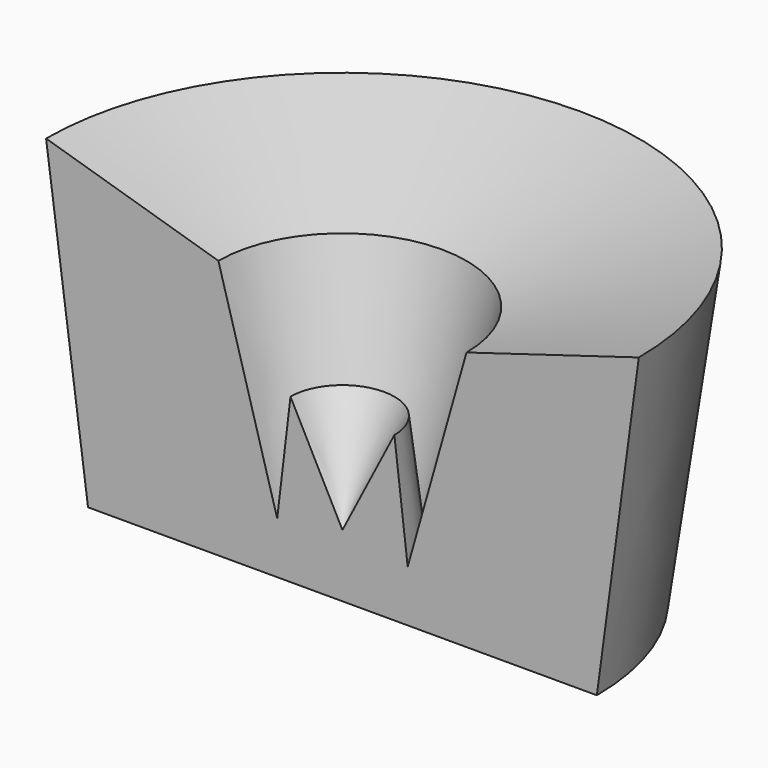
from build123d import *

# Parameters (mm, degrees)
F1_ANGLE = 180


# Not quite as in the source:
# - the program builds the solid bodies; features that only make, move or delete a surface that nothing else refers to are left out


with BuildPart() as f1:
    # F0 (on Front) → F1 (revolve)
    with BuildSketch(Plane.XZ):
        Polygon((12.4851092696, 39.2489619553), (0, 15.0755345821), (0, 0), (61.1490756273, 0), (71.2305568159, 74.7646316886), (29.8195946962, 62.3483546078), (15.6820116428, 12.4102499136), align=None)
    revolve(axis=Axis((0, 0, 7.5377672911), (0, 0, 1)), revolution_arc=F1_ANGLE)


solid = f1.part
